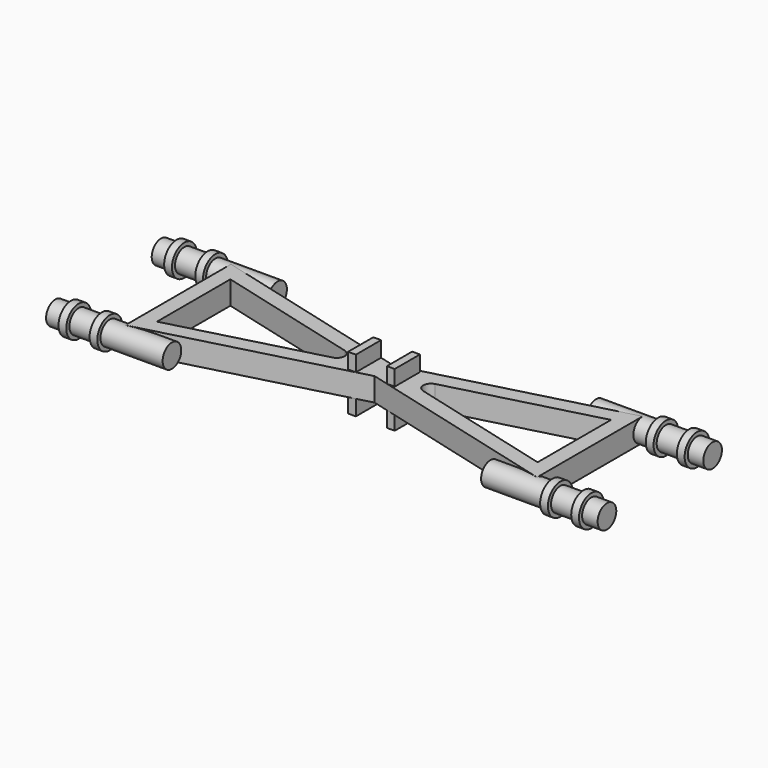
from build123d import *

# Parameters (mm, degrees)
F1_DEPTH = 1.5
F3_DEPTH = 3.001
F4_R     = 1
F7_W     = 1
F7_H     = 4.0566037736
F8_DEPTH = 3.5


# Not quite as in the source:
# - a feature names something its author has since deleted; it is built from what else it names


with BuildPart() as f1:
    # F0 (on Top) → F1 (new body, symmetric)
    with BuildSketch(Plane.XY):
        Polygon((0, 1.5), (-26.5, 8.5), (-26.5, 0), (-26.5, -8.5), (0, -1.5), (26.5, -8.5), (26.5, 0), (26.5, 8.5), align=None)
    extrude(amount=F1_DEPTH, both=True)

    # F2 (on face) → F3 (cut, through all)
    with BuildSketch(Plane.XY.offset(1.5)):
        Polygon((-24.5, 5.9030988568), (-24.5, 0), (-24.5, -5.9030988568), (-2.1525543278, 0), align=None)
        Polygon((24.5, 0), (24.5, 5.9030988568), (2.1525543278, 0), (24.5, -5.9030988568), align=None)
    extrude(amount=-F3_DEPTH, mode=Mode.SUBTRACT)

    # F4
    f4_edges = [f1.edges().sort_by_distance(p)[0] for p in [
        (-2.152554, 0, 0),
        (2.152554, 0, 0),
    ]]
    fillet(f4_edges, radius=F4_R)

    # F5 (on Top) → F6 (revolve)
    with BuildSketch(Plane.XY):
        Polygon((20.5, 8.5), (35.5, 8.5), (35.5, 10), (33.5, 10), (33.5, 10.5), (32.5, 10.5), (32.5, 10), (29.5, 10), (29.5, 10.5), (28.5, 10.5), (28.5, 10), (20.5, 10), align=None)
    revolve(axis=Axis((28, 8.5, 0), (1, 0, 0)))

    # F7 (on Top) → F8 (join, symmetric)
    with BuildSketch(Plane.XY):
        with Locations((-2.5, 0)):
            Rectangle(F7_W, F7_H)
    extrude(amount=F8_DEPTH, both=True)

    # F9: F1 across plane


with BuildPart() as f1_1:
    add(f1.part)
    add(f1.part.mirror(Plane.YZ))

    # F10: F1 across plane


with BuildPart() as f1_2:
    add(f1_1.part)
    add(f1_1.part.mirror(Plane.XZ))


solid = f1_2.part
